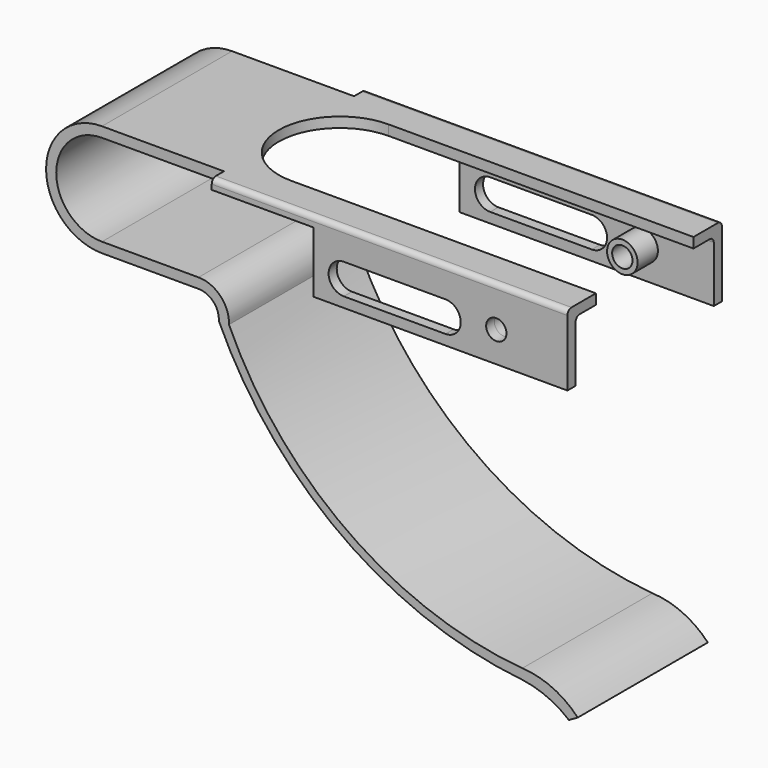
from build123d import *

# Parameters (mm, degrees)
F1_DEPTH  = 16
F2_W      = 70
F2_H      = 3
F3_DEPTH  = 2
F4_W      = 50
F4_H      = 12
F5_DEPTH  = 2
F6_R      = 1
F9_DEPTH  = 2
F11_DEPTH = 38.001
F13_D     = 4
F14_R     = 3
F14_R_2   = 2
F15_DEPTH = 5


# Not quite as in the source:
# - a pattern or mirror of a feature is missing from the dataset's text; its kind, count and spacing are read off the source's solid


with BuildPart() as f1:
    # F0 (on Front) → F1 (new body)
    with BuildSketch(Plane.XZ):
        with BuildLine():
            Line((46.2855722755, 5.7414249778), (-47.7144277245, 5.7414249778))
            ThreePointArc((-47.7144277245, 5.7414249778), (-58.7144277245, -5.2585750222), (-47.7144277245, -16.2585750222))
            Line((-47.7144277245, -16.2585750222), (-28.7144277245, -16.2585750222))
            ThreePointArc((-28.7144277245, -16.2585750222), (-25.7968307423, -17.5210599177), (-24.7197856057, -20.5120821569))
            ThreePointArc((-24.7197856057, -20.5120821569), (-0.5386319719, -49.8206199667), (35.0020481502, -63.2585750222))
            ThreePointArc((35.0020481502, -63.2585750222), (39.8678360266, -64.6074545818), (44.1721712505, -67.2471640366))
            Line((44.1721712505, -67.2471640366), (45.9107602648, -66.2585750222))
            ThreePointArc((45.9107602648, -66.2585750222), (40.9429054682, -62.6971545828), (35.0020481502, -61.2585750222))
            ThreePointArc((35.0020481502, -61.2585750222), (0.6230450398, -48.7022972109), (-22.7197856057, -20.5120821569))
            ThreePointArc((-22.7197856057, -20.5120821569), (-24.3830859689, -16.1065299122), (-28.7144277245, -14.2585750222))
            Line((-28.7144277245, -14.2585750222), (-47.7144277245, -14.2585750222))
            ThreePointArc((-47.7144277245, -14.2585750222), (-56.7144277245, -5.2585750222), (-47.7144277245, 3.7414249778))
            Line((-47.7144277245, 3.7414249778), (46.2855722755, 3.7414249778))
            Line((46.2855722755, 3.7414249778), (46.2855722755, 5.7414249778))
        make_face()
    extrude(amount=F1_DEPTH)

    # F2 (on face) → F3 (join)
    with BuildSketch(Plane.XY.offset(5.7414249778)):
        with Locations((11.2855722755, -17.5)):
            Rectangle(F2_W, F2_H)
    extrude(amount=-F3_DEPTH)

    # F4 (on face) → F5 (join)
    with BuildSketch(Plane.XZ.offset(19)):
        with Locations((21.2855722755, -2.2585750222)):
            Rectangle(F4_W, F4_H)
    extrude(amount=-F5_DEPTH)

    # F6
    f6_edges = [f1.edges().sort_by_distance(p)[0] for p in [
        (11.285572, -19, 5.741425),
        (21.285572, -17, 3.741425),
    ]]
    fillet(f6_edges, radius=F6_R)

    # F7: F1 across plane


with BuildPart() as f1_1:
    add(f1.part)
    add(f1.part.mirror(Plane.XZ))

    # F8 (on face) → F9 (cut)
    with BuildSketch(Plane.XY.offset(5.7414249778)):
        with BuildLine():
            Line((46.2855722755, 12), (-13.7144277245, 12))
            ThreePointArc((-13.7144277245, 12), (-25.7144277245, 0), (-13.7144277245, -12))
            Line((-13.7144277245, -12), (46.2855722755, -12))
            Line((46.2855722755, -12), (46.2855722755, 12))
        make_face()
    extrude(amount=-F9_DEPTH, mode=Mode.SUBTRACT)

    # F10 (on face) → F11 (cut, through all)
    with BuildSketch(Plane.XZ.offset(19)):
        with BuildLine():
            ThreePointArc((2.2855722755, -0.2585750222), (-0.7144277245, -3.2585750222), (2.2855722755, -6.2585750222))
            Line((2.2855722755, -6.2585750222), (22.2855722755, -6.2585750222))
            ThreePointArc((22.2855722755, -6.2585750222), (25.2855722755, -3.2585750222), (22.2855722755, -0.2585750222))
            Line((22.2855722755, -0.2585750222), (2.2855722755, -0.2585750222))
        make_face()
    extrude(amount=-F11_DEPTH, mode=Mode.SUBTRACT)

    # F13 (through all)
    with Locations(Plane.XZ.offset(19)):
        with Locations((32.2855722755, -2.2585750222)):
            Hole(F13_D / 2)

    # F14 (on face) → F15 (join)
    with BuildSketch(Plane(origin=(0, -17, 0), x_dir=(-1, 0, 0), z_dir=(0, 1, 0))):
        with Locations((-32.2855722755, -2.2585750222)):
            Circle(F14_R)
        with Locations((-32.2855722755, -2.2585750222)):
            Circle(F14_R_2, mode=Mode.SUBTRACT)
    f15 = extrude(amount=F15_DEPTH)

    # F15_copies: F15 across plane
    add(f15.mirror(Plane.ZX))


solid = f1_1.part
